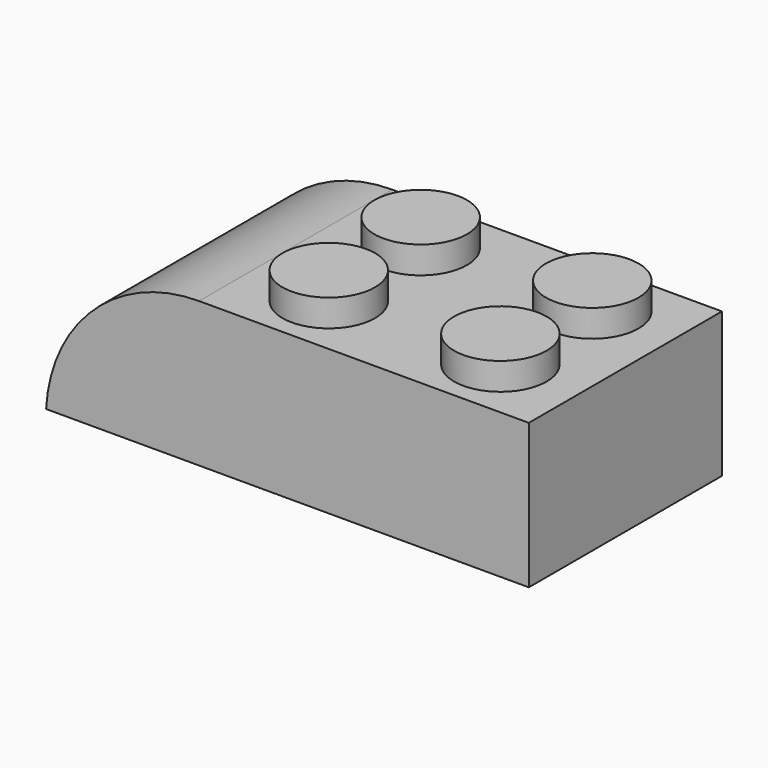
from build123d import *

# Parameters (mm, degrees)
F0_W        = 32
F0_H        = 16
F1_DEPTH    = 9.6
F2_T1_DEPTH = 66.7227759493
F3_R        = 3.0688775333
F4_DEPTH    = 1.8


# Not quite as in the source:
# - a fillet or chamfer that OpenCascade refuses, or shapes differently, is made with other operations: its cross-section is extruded or revolved along the edge and cut away or added
# - a feature names something its author has since deleted; it is built from what else it names


with BuildPart() as f1:
    # F0 (on Top) → F1 (new body)
    with BuildSketch(Plane.XY):
        with Locations((-16, 8)):
            Rectangle(F0_W, F0_H)
    extrude(amount=F1_DEPTH)

    # F2: fillet of radius 10.16 on 1 edges, made by hand

    # F2_s2 → F2_t1 (cut)
    with BuildSketch(Plane.XZ.offset(-41.3613879746)):
        with BuildLine():
            ThreePointArc((-32, 0), (-28.8388537198, 6.819539281), (-21.8554448101, 9.6))
            Line((-21.8554448101, 9.6), (-32, 9.6))
            Line((-32, 9.6), (-32, 0))
        make_face()
    extrude(amount=F2_T1_DEPTH, mode=Mode.SUBTRACT)

    # F3 (on face) → F4 (join)
    with BuildSketch(Plane.XY.offset(9.6)):
        with Locations((-16.6150905888, 11.8076978251)):
            Circle(F3_R)
        with Locations((-5.2403542213, 11.8076978251)):
            Circle(F3_R)
        with Locations((-16.6150905888, 4.1923021749)):
            Circle(F3_R)
        with Locations((-5.2403542213, 4.1923021749)):
            Circle(F3_R)
    extrude(amount=F4_DEPTH)


solid = f1.part
